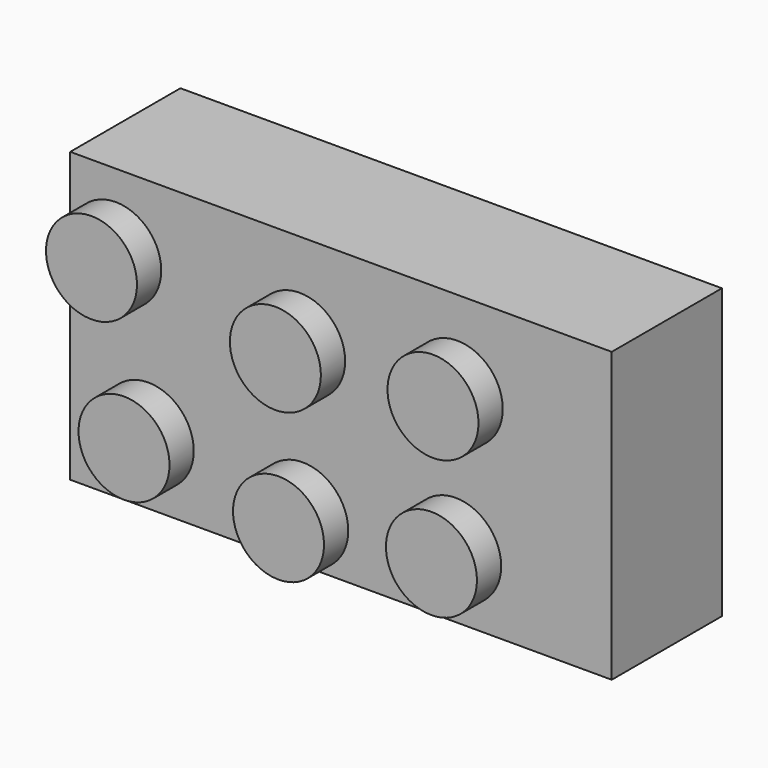
from build123d import *
from build123d import SkipClean  # not in build123d's __all__

# Parameters (mm, degrees)
F0_W         = 99.8685993254
F0_H         = 53.244067356
F1_DEPTH     = 25.4
F2_R         = 8.3909074383
F3_DEPTH     = 5.588
F4_T         = 0.254
F4_T6_ANGLE  = 90.000000253
F4_T8_ANGLE  = 269.999999749
F4_T12_ANGLE = 180.000000001
F4_T14_ANGLE = 180.000000001


# Not quite as in the source:
# - a shell that OpenCascade refuses in one call is made with other operations: the cavity is built on its own and cut out


with BuildPart() as f1:
    # F0 (on Front) → F1 (new body)
    with BuildSketch(Plane.XZ):
        with Locations((2.4463478476, -0.7195146754)):
            Rectangle(F0_W, F0_H)
    extrude(amount=F1_DEPTH)

    # F2 (on face) → F3 (join)
    with BuildSketch(Plane.XZ.offset(25.4)):
        with Locations((-5.1805051044, 8.3909074383)):
            Circle(F2_R)
        with Locations((23.8878745586, 10.0732017308)):
            Circle(F2_R)
        with Locations((23.600069806, -15.5415115878)):
            Circle(F2_R)
        with Locations((-4.6048937365, -18.9506409151)):
            Circle(F2_R)
        with Locations((-33.0976620317, -15.2537049726)):
            Circle(F2_R)
        with Locations((-39.0970443768, 12.0878415182)):
            Circle(F2_R)
    extrude(amount=F3_DEPTH)

    # F4: shell of thickness 0.254, made by hand


with BuildPart() as f4_core1:
    # F4_t2: copy of F1
    add(f1.part, clean=False)

    # the walls: a layer under each face that stays
    f4_faces = [f4_core1.faces().sort_by_distance(p)[0] for p in [
        (-47.4879518151, -12.7, -0.7195146754),
        (2.4463478476, -12.7, 25.9025190026),
        (2.4463478476, -12.7, -27.3415483534),
        (2.4463478476, -25.4, -0.7195146754),
        (52.3806475103, -12.7, -0.7195146754),
        (-41.48856947, -28.194, -15.2537049726),
        (-12.9958011749, -28.194, -18.9506409151),
        (15.2091623677, -28.194, -15.5415115878),
        (-47.4879518151, -28.194, 12.0878415182),
        (-13.5714125427, -28.194, 8.3909074383),
        (15.4969671202, -28.194, 10.0732017308),
        (-33.0976620317, -30.988, -15.2537049726),
        (-4.6048937365, -30.988, -18.9506409151),
        (23.600069806, -30.988, -15.5415115878),
        (-39.0970443768, -30.988, 12.0878415182),
        (-5.1805051044, -30.988, 8.3909074383),
        (23.8878745586, -30.988, 10.0732017308),
    ]]
    thicken(f4_faces, amount=-F4_T, mode=Mode.SUBTRACT)

    # F4_s3 → F4_t4 (revolve, cut)
    with BuildSketch(Plane.XY.offset(-15.2537049726)):
        Polygon((-24.7042145933, -25.40254), (-24.7067545933, -25.146), (-24.9607545933, -25.146), (-24.9607545933, -25.4), align=None)
    revolve(axis=Axis((-33.0976620317, -25.4, -15.2537049726), (0, -1, 0)), mode=Mode.SUBTRACT)

    # F4_s5 → F4_t6 (revolve, cut)
    with BuildSketch(Plane.YZ.offset(-4.6048937365)):
        Polygon((-25.40254, -27.3440883534), (-25.146, -27.3415483534), (-25.146, -27.0875483534), (-25.4, -27.0875483534), align=None)
    revolve(axis=Axis((-4.6048937365, -25.4, -18.9506409151), (0, -1, 0)), revolution_arc=F4_T6_ANGLE, mode=Mode.SUBTRACT)

    # F4_s7 → F4_t8 (revolve, cut)
    with BuildSketch(Plane.XY.offset(-18.9506409151)):
        Polygon((3.7885537018, -25.40254), (3.7860137018, -25.146), (3.5320137018, -25.146), (3.5320137018, -25.4), align=None)
    revolve(axis=Axis((-4.6048937365, -25.4, -18.9506409151), (0, -1, 0)), revolution_arc=F4_T8_ANGLE, mode=Mode.SUBTRACT)

    # F4_s9 → F4_t10 (revolve, cut)
    with BuildSketch(Plane.XY.offset(-15.5415115878)):
        Polygon((31.9935172443, -25.40254), (31.9909772443, -25.146), (31.7369772443, -25.146), (31.7369772443, -25.4), align=None)
    revolve(axis=Axis((23.600069806, -25.4, -15.5415115878), (0, -1, 0)), mode=Mode.SUBTRACT)

    # F4_s11 → F4_t12 (revolve, cut)
    with BuildSketch(Plane.XY.offset(12.0878415182)):
        Polygon((-47.4904918151, -25.40254), (-47.4879518151, -25.146), (-47.2339518151, -25.146), (-47.2339518151, -25.4), align=None)
    with SkipClean():  # cleaning this boolean's faces spoils the solid; the shape is the same uncleaned
        revolve(axis=Axis((-39.0970443768, -25.4, 12.0878415182), (0, -1, 0)), revolution_arc=F4_T12_ANGLE, mode=Mode.SUBTRACT)

    # F4_s13 → F4_t14 (revolve, cut)
    with BuildSketch(Plane.XY.offset(12.0878415182)):
        Polygon((-30.7035969385, -25.40254), (-30.7061369385, -25.146), (-30.9601369385, -25.146), (-30.9601369385, -25.4), align=None)
    revolve(axis=Axis((-39.0970443768, -25.4, 12.0878415182), (0, -1, 0)), revolution_arc=F4_T14_ANGLE, mode=Mode.SUBTRACT)

    # F4_s15 → F4_t16 (revolve, cut)
    with BuildSketch(Plane.XY.offset(8.3909074383)):
        Polygon((3.212942334, -25.40254), (3.210402334, -25.146), (2.956402334, -25.146), (2.956402334, -25.4), align=None)
    revolve(axis=Axis((-5.1805051044, -25.4, 8.3909074383), (0, -1, 0)), mode=Mode.SUBTRACT)

    # F4_s17 → F4_t18 (revolve, cut)
    with BuildSketch(Plane.XY.offset(10.0732017308)):
        Polygon((32.2813219969, -25.40254), (32.2787819969, -25.146), (32.0247819969, -25.146), (32.0247819969, -25.4), align=None)
    revolve(axis=Axis((23.8878745586, -25.4, 10.0732017308), (0, -1, 0)), mode=Mode.SUBTRACT)


with BuildPart() as f1_1:
    add(f1.part, clean=False)

    # what is left inside the walls is the cavity
    f4_cavity = [f4_core1.part.solids().sort_by_distance(p)[0] for p in [
        (2.446348, -0.00254, -9.508859),
    ]]
    add(f4_cavity, mode=Mode.SUBTRACT)


solid = f1_1.part
